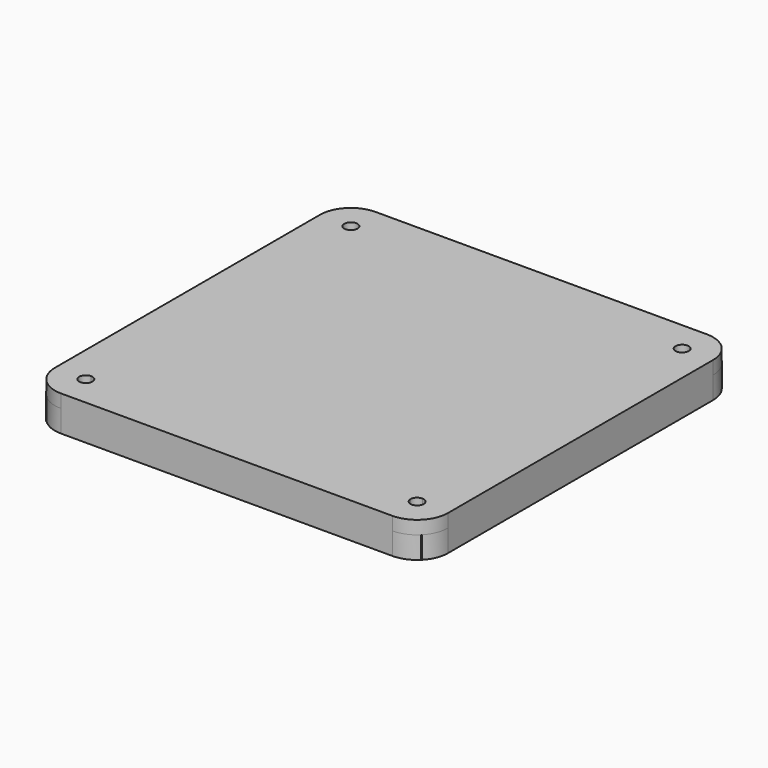
from build123d import *

# Parameters (mm, degrees)
F1_DEPTH = 3
F2_R     = 1.5
F2_W     = 1
F2_H     = 15
F2_W_2   = 9
F2_H_2   = 1
F2_W_3   = 10
F2_H_3   = 10
F2_W_4   = 16
F2_W_5   = 15
F3_DEPTH = 5


with BuildPart() as f1:
    # F0 (on Top) → F1 (new body)
    with BuildSketch(Plane.XY):
        with BuildLine():
            ThreePointArc((-37.5, 44.5), (-32.5502525317, 42.4497474683), (-30.5, 37.5))
            Line((-30.5, 37.5), (30.5, 37.5))
            ThreePointArc((30.5, 37.5), (32.5502525317, 42.4497474683), (37.5, 44.5))
            Line((37.5, 44.5), (-37.5, 44.5))
        make_face()
        with BuildLine():
            Line((30.5, -37.5), (-30.5, -37.5))
            ThreePointArc((-30.5, -37.5), (-32.550252511, -42.4497474476), (-37.4999999416, -44.5))
            Line((-37.4999999416, -44.5), (37.5, -44.5))
            ThreePointArc((37.5, -44.5), (32.5502525317, -42.4497474683), (30.5, -37.5))
        make_face()
        with BuildLine():
            ThreePointArc((44.5, 37.5), (42.4497474683, 32.5502525317), (37.5, 30.5))
            Line((37.5, 30.5), (37.5, -30.5))
            ThreePointArc((37.5, -30.5), (42.4497474683, -32.5502525317), (44.5, -37.5))
            Line((44.5, -37.5), (44.5, 37.5))
        make_face()
        with BuildLine():
            Line((-37.5, -30.5), (-37.5, 30.5))
            ThreePointArc((-37.5, 30.5), (-42.4497474683, 32.5502525317), (-44.5, 37.5))
            Line((-44.5, 37.5), (-44.5, -37.4999999639))
            ThreePointArc((-44.5, -37.4999999639), (-42.4497474555, -32.5502525189), (-37.5, -30.5))
        make_face()
        with BuildLine():
            ThreePointArc((37.5, 44.5), (32.5502525317, 42.4497474683), (30.5, 37.5))
            Line((30.5, 37.5), (36, 37.5))
            ThreePointArc((36, 37.5), (37.5, 39), (39, 37.5))
            ThreePointArc((39, 37.5), (38.5606601718, 36.4393398282), (37.5, 36))
            Line((37.5, 36), (37.5, 30.5))
            ThreePointArc((37.5, 30.5), (42.4497474683, 32.5502525317), (44.5, 37.5))
            ThreePointArc((44.5, 37.5), (42.4497474683, 42.4497474683), (37.5, 44.5))
        make_face()
        with BuildLine():
            Line((-36, 37.5), (-30.5, 37.5))
            ThreePointArc((-30.5, 37.5), (-32.5502525317, 42.4497474683), (-37.5, 44.5))
            ThreePointArc((-37.5, 44.5), (-42.4497474683, 42.4497474683), (-44.5, 37.5))
            ThreePointArc((-44.5, 37.5), (-42.4497474683, 32.5502525317), (-37.5, 30.5))
            Line((-37.5, 30.5), (-37.5, 36))
            ThreePointArc((-37.5, 36), (-38.5606601718, 38.5606601718), (-36, 37.5))
        make_face()
        with BuildLine():
            ThreePointArc((44.5, -37.5), (42.4497474683, -32.5502525317), (37.5, -30.5))
            Line((37.5, -30.5), (37.5, -36))
            ThreePointArc((37.5, -36), (38.5606601718, -36.4393398282), (39, -37.5))
            ThreePointArc((39, -37.5), (37.5, -39), (36, -37.5))
            Line((36, -37.5), (30.5, -37.5))
            ThreePointArc((30.5, -37.5), (32.5502525317, -42.4497474683), (37.5, -44.5))
            ThreePointArc((37.5, -44.5), (42.4497474683, -42.4497474683), (44.5, -37.5))
        make_face()
        with BuildLine():
            Line((-37.5, -36), (-37.5, -30.5))
            ThreePointArc((-37.5, -30.5), (-42.4497474555, -32.5502525189), (-44.5, -37.4999999639))
            ThreePointArc((-44.5, -37.4999999639), (-42.4497474604, -42.4497474762), (-37.4999999416, -44.5))
            ThreePointArc((-37.4999999416, -44.5), (-32.550252511, -42.4497474476), (-30.5, -37.5))
            Line((-30.5, -37.5), (-36, -37.5))
            ThreePointArc((-36, -37.5), (-38.5606601718, -38.5606601718), (-37.5, -36))
        make_face()
        with BuildLine():
            Line((30.5, 37.5), (-30.5, 37.5))
            ThreePointArc((-30.5, 37.5), (-32.5502525317, 32.5502525317), (-37.5, 30.5))
            Line((-37.5, 30.5), (-37.5, -30.5))
            ThreePointArc((-37.5, -30.5), (-32.5502525317, -32.5502525317), (-30.5, -37.5))
            Line((-30.5, -37.5), (30.5, -37.5))
            ThreePointArc((30.5, -37.5), (32.5502525317, -32.5502525317), (37.5, -30.5))
            Line((37.5, -30.5), (37.5, 30.5))
            ThreePointArc((37.5, 30.5), (32.5502525317, 32.5502525317), (30.5, 37.5))
        make_face()
        with BuildLine():
            ThreePointArc((-37.5, 30.5), (-32.5502525317, 32.5502525317), (-30.5, 37.5))
            Line((-30.5, 37.5), (-36, 37.5))
            ThreePointArc((-36, 37.5), (-36.4393398282, 36.4393398282), (-37.5, 36))
            Line((-37.5, 36), (-37.5, 30.5))
        make_face()
        with BuildLine():
            Line((36, 37.5), (30.5, 37.5))
            ThreePointArc((30.5, 37.5), (32.5502525317, 32.5502525317), (37.5, 30.5))
            Line((37.5, 30.5), (37.5, 36))
            ThreePointArc((37.5, 36), (36.4393398282, 36.4393398282), (36, 37.5))
        make_face()
        with BuildLine():
            Line((37.5, -36), (37.5, -30.5))
            ThreePointArc((37.5, -30.5), (32.5502525317, -32.5502525317), (30.5, -37.5))
            Line((30.5, -37.5), (36, -37.5))
            ThreePointArc((36, -37.5), (36.4393398282, -36.4393398282), (37.5, -36))
        make_face()
        with BuildLine():
            ThreePointArc((-30.5, -37.5), (-32.5502525317, -32.5502525317), (-37.5, -30.5))
            Line((-37.5, -30.5), (-37.5, -36))
            ThreePointArc((-37.5, -36), (-36.4393398282, -36.4393398282), (-36, -37.5))
            Line((-36, -37.5), (-30.5, -37.5))
        make_face()
    extrude(amount=F1_DEPTH)

    # F2 (on face) → F3 (join)
    with BuildSketch(Plane(origin=(0, 0, 0), x_dir=(1, 0, 0), z_dir=(0, 0, -1))):
        with BuildLine():
            Line((42.5, 42.3989794856), (42.5, 42.5))
            Line((42.5, 42.5), (42.3989794856, 42.5))
            ThreePointArc((42.3989794856, 42.5), (42.4497474683, 42.4497474683), (42.5, 42.3989794856))
        make_face()
        with BuildLine():
            ThreePointArc((42.5, 42.3989794856), (42.4497474683, 42.4497474683), (42.3989794856, 42.5))
            Line((42.3989794856, 42.5), (37.5, 42.5))
            ThreePointArc((37.5, 42.5), (41.0355339059, 41.0355339059), (42.5, 37.5))
            Line((42.5, 37.5), (42.5, 42.3989794856))
        make_face()
        with BuildLine():
            Line((37.5, 42.5), (42.3989794856, 42.5))
            ThreePointArc((42.3989794856, 42.5), (40.1457513111, 43.9807406984), (37.5, 44.5))
            ThreePointArc((37.5, 44.5), (34.8542486889, 43.9807406984), (32.6010205144, 42.5))
            Line((32.6010205144, 42.5), (37.5, 42.5))
        make_face()
        with BuildLine():
            ThreePointArc((44.5, 37.5), (43.9807406984, 40.1457513111), (42.5, 42.3989794856))
            Line((42.5, 42.3989794856), (42.5, 37.5))
            Line((42.5, 37.5), (42.5, 32.6010205144))
            ThreePointArc((42.5, 32.6010205144), (43.9807406984, 34.8542486889), (44.5, 37.5))
        make_face()
        with BuildLine():
            ThreePointArc((42.5, 37.5), (33.9644660941, 33.9644660941), (37.5, 42.5))
            Line((37.5, 42.5), (32.6010205144, 42.5))
            ThreePointArc((32.6010205144, 42.5), (32.5502525317, 32.5502525317), (42.5, 32.6010205144))
            Line((42.5, 32.6010205144), (42.5, 37.5))
        make_face()
        with BuildLine():
            ThreePointArc((42.5, 37.5), (41.0355339059, 41.0355339059), (37.5, 42.5))
            ThreePointArc((37.5, 42.5), (33.9644660941, 33.9644660941), (42.5, 37.5))
        make_face()
        with Locations((37.5, 37.5)):
            Circle(F2_R, mode=Mode.SUBTRACT)
        with BuildLine():
            ThreePointArc((32.6010205144, 42.5), (34.8542486889, 43.9807406984), (37.5, 44.5))
            Line((37.5, 44.5), (-37.4999999416, 44.5))
            ThreePointArc((-37.4999999416, 44.5), (-34.8542486619, 43.9807406874), (-32.6010205144, 42.5))
            Line((-32.6010205144, 42.5), (32.6010205144, 42.5))
        make_face()
        with BuildLine():
            Line((44.5, -37.5), (44.5, 37.5))
            ThreePointArc((44.5, 37.5), (43.9807406984, 34.8542486889), (42.5, 32.6010205144))
            Line((42.5, 32.6010205144), (42.5, -32.6010205144))
            ThreePointArc((42.5, -32.6010205144), (43.9807406984, -34.8542486889), (44.5, -37.5))
        make_face()
        with BuildLine():
            ThreePointArc((-32.6010205144, 42.5), (-34.8542486619, 43.9807406874), (-37.4999999416, 44.5))
            ThreePointArc((-37.4999999416, 44.5), (-40.145751284, 43.9807407095), (-42.3989794856, 42.5))
            Line((-42.3989794856, 42.5), (-37.5, 42.5))
            Line((-37.5, 42.5), (-32.6010205144, 42.5))
        make_face()
        with BuildLine():
            ThreePointArc((42.5, -42.3989794856), (43.9807406984, -40.1457513111), (44.5, -37.5))
            ThreePointArc((44.5, -37.5), (43.9807406984, -34.8542486889), (42.5, -32.6010205144))
            Line((42.5, -32.6010205144), (42.5, -37.5))
            Line((42.5, -37.5), (42.5, -42.3989794856))
        make_face()
        with BuildLine():
            ThreePointArc((-30.5, 37.5), (-31.0465956117, 40.2117470016), (-32.6010205144, 42.5))
            Line((-32.6010205144, 42.5), (-37.5, 42.5))
            ThreePointArc((-37.5, 42.5), (-33.9644660941, 41.0355339059), (-32.5, 37.5))
            ThreePointArc((-32.5, 37.5), (-37.5, 32.5), (-42.5, 37.5))
            Line((-42.5, 37.5), (-42.5, 32.6010205144))
            ThreePointArc((-42.5, 32.6010205144), (-34.8542486889, 31.0192593016), (-30.5, 37.5))
        make_face()
        with BuildLine():
            ThreePointArc((-42.5, 42.3989794856), (-42.4497474683, 42.4497474683), (-42.3989794856, 42.5))
            Line((-42.3989794856, 42.5), (-42.5, 42.5))
            Line((-42.5, 42.5), (-42.5, 42.3989794856))
        make_face()
        with BuildLine():
            Line((-37.5, 42.5), (-42.3989794856, 42.5))
            ThreePointArc((-42.3989794856, 42.5), (-42.4497474683, 42.4497474683), (-42.5, 42.3989794856))
            Line((-42.5, 42.3989794856), (-42.5, 37.5))
            ThreePointArc((-42.5, 37.5), (-41.0355339059, 41.0355339059), (-37.5, 42.5))
        make_face()
        with BuildLine():
            Line((42.5, -37.5), (42.5, -32.6010205144))
            ThreePointArc((42.5, -32.6010205144), (32.5502525317, -32.5502525317), (32.6010205144, -42.5))
            Line((32.6010205144, -42.5), (37.5, -42.5))
            ThreePointArc((37.5, -42.5), (33.9644660941, -33.9644660941), (42.5, -37.5))
        make_face()
        with BuildLine():
            ThreePointArc((42.3989794856, -42.5), (42.4497474683, -42.4497474683), (42.5, -42.3989794856))
            Line((42.5, -42.3989794856), (42.5, -37.5))
            ThreePointArc((42.5, -37.5), (41.0355339059, -41.0355339059), (37.5, -42.5))
            Line((37.5, -42.5), (42.3989794856, -42.5))
        make_face()
        with BuildLine():
            Line((42.5, -42.5), (42.5, -42.3989794856))
            ThreePointArc((42.5, -42.3989794856), (42.4497474683, -42.4497474683), (42.3989794856, -42.5))
            Line((42.3989794856, -42.5), (42.5, -42.5))
        make_face()
        with BuildLine():
            ThreePointArc((-32.5, 37.5), (-33.9644660941, 41.0355339059), (-37.5, 42.5))
            ThreePointArc((-37.5, 42.5), (-41.0355339059, 41.0355339059), (-42.5, 37.5))
            ThreePointArc((-42.5, 37.5), (-37.5, 32.5), (-32.5, 37.5))
        make_face()
        with Locations((-37.5, 37.5)):
            Circle(F2_R, mode=Mode.SUBTRACT)
        with BuildLine():
            Line((-42.5, 37.5), (-42.5, 42.3989794856))
            ThreePointArc((-42.5, 42.3989794856), (-43.9807407052, 40.1457512943), (-44.5, 37.4999999639))
            ThreePointArc((-44.5, 37.4999999639), (-43.9807406916, 34.8542486722), (-42.5, 32.6010205144))
            Line((-42.5, 32.6010205144), (-42.5, 37.5))
        make_face()
        with BuildLine():
            ThreePointArc((37.5, -42.5), (41.0355339059, -41.0355339059), (42.5, -37.5))
            ThreePointArc((42.5, -37.5), (33.9644660941, -33.9644660941), (37.5, -42.5))
        make_face()
        with Locations((37.5, -37.5)):
            Circle(F2_R, mode=Mode.SUBTRACT)
        with BuildLine():
            ThreePointArc((37.5, -44.5), (34.8542486889, -43.9807406984), (32.6010205144, -42.5))
            Line((32.6010205144, -42.5), (-32.6010205144, -42.5))
            ThreePointArc((-32.6010205144, -42.5), (-34.8542486889, -43.9807406984), (-37.5, -44.5))
            Line((-37.5, -44.5), (37.5, -44.5))
        make_face()
        with BuildLine():
            Line((37.5, -42.5), (32.6010205144, -42.5))
            ThreePointArc((32.6010205144, -42.5), (34.8542486889, -43.9807406984), (37.5, -44.5))
            ThreePointArc((37.5, -44.5), (40.1457513111, -43.9807406984), (42.3989794856, -42.5))
            Line((42.3989794856, -42.5), (37.5, -42.5))
        make_face()
        with BuildLine():
            Line((-42.5, -32.6010205144), (-42.5, 32.6010205144))
            ThreePointArc((-42.5, 32.6010205144), (-43.9807406916, 34.8542486722), (-44.5, 37.4999999639))
            Line((-44.5, 37.4999999639), (-44.5, -37.5))
            ThreePointArc((-44.5, -37.5), (-43.9807406984, -34.8542486889), (-42.5, -32.6010205144))
        make_face()
        with BuildLine():
            ThreePointArc((-37.5, -44.5), (-34.8542486889, -43.9807406984), (-32.6010205144, -42.5))
            Line((-32.6010205144, -42.5), (-37.5, -42.5))
            Line((-37.5, -42.5), (-42.3989794856, -42.5))
            ThreePointArc((-42.3989794856, -42.5), (-40.1457513111, -43.9807406984), (-37.5, -44.5))
        make_face()
        with BuildLine():
            Line((-37.5, -42.5), (-32.6010205144, -42.5))
            ThreePointArc((-32.6010205144, -42.5), (-31.0465956117, -40.2117470016), (-30.5, -37.5))
            ThreePointArc((-30.5, -37.5), (-34.8542486889, -31.0192593016), (-42.5, -32.6010205144))
            Line((-42.5, -32.6010205144), (-42.5, -37.5))
            ThreePointArc((-42.5, -37.5), (-37.5, -32.5), (-32.5, -37.5))
            ThreePointArc((-32.5, -37.5), (-33.9644660941, -41.0355339059), (-37.5, -42.5))
        make_face()
        with BuildLine():
            Line((-42.5, -37.5), (-42.5, -32.6010205144))
            ThreePointArc((-42.5, -32.6010205144), (-43.9807406984, -34.8542486889), (-44.5, -37.5))
            ThreePointArc((-44.5, -37.5), (-43.9807406984, -40.1457513111), (-42.5, -42.3989794856))
            Line((-42.5, -42.3989794856), (-42.5, -37.5))
        make_face()
        with BuildLine():
            Line((-42.3989794856, -42.5), (-37.5, -42.5))
            ThreePointArc((-37.5, -42.5), (-41.0355339059, -41.0355339059), (-42.5, -37.5))
            Line((-42.5, -37.5), (-42.5, -42.3989794856))
            ThreePointArc((-42.5, -42.3989794856), (-42.4497474683, -42.4497474683), (-42.3989794856, -42.5))
        make_face()
        with BuildLine():
            ThreePointArc((-42.5, -37.5), (-41.0355339059, -41.0355339059), (-37.5, -42.5))
            ThreePointArc((-37.5, -42.5), (-33.9644660941, -41.0355339059), (-32.5, -37.5))
            ThreePointArc((-32.5, -37.5), (-37.5, -32.5), (-42.5, -37.5))
        make_face()
        with Locations((-37.5, -37.5)):
            Circle(F2_R, mode=Mode.SUBTRACT)
        with BuildLine():
            ThreePointArc((-42.3989794856, -42.5), (-42.4497474683, -42.4497474683), (-42.5, -42.3989794856))
            Line((-42.5, -42.3989794856), (-42.5, -42.5))
            Line((-42.5, -42.5), (-42.3989794856, -42.5))
        make_face()
        with Locations((0, 30)):
            Rectangle(F2_W, F2_H)
        with Locations((5, 22)):
            Rectangle(F2_W_2, F2_H_2)
        with Locations((0, 22)):
            Rectangle(F2_W, F2_H_2)
        with Locations((-5.5, 22)):
            Rectangle(F2_W_3, F2_H_2)
        with Locations((0, 16.5)):
            Rectangle(F2_W, F2_H_3)
        with Locations((10, 30)):
            Rectangle(F2_W, F2_H)
        with Locations((10, 22)):
            Rectangle(F2_W, F2_H_2)
        with Locations((-11, 22)):
            Rectangle(F2_W, F2_H_2)
        with Locations((-11, 30)):
            Rectangle(F2_W, F2_H)
        with Locations((5, 11)):
            Rectangle(F2_W_2, F2_H_2)
        with Locations((0, 11)):
            Rectangle(F2_W, F2_H_2)
        with Locations((10, 16.5)):
            Rectangle(F2_W, F2_H_3)
        with Locations((15.5, 22)):
            Rectangle(F2_W_3, F2_H_2)
        with Locations((-5.5, 11)):
            Rectangle(F2_W_3, F2_H_2)
        with Locations((-11, 16.5)):
            Rectangle(F2_W, F2_H_3)
        with Locations((-16.5, 22)):
            Rectangle(F2_W_3, F2_H_2)
        with Locations((0, 5.5)):
            Rectangle(F2_W, F2_H_3)
        with Locations((10, 11)):
            Rectangle(F2_W, F2_H_2)
        with Locations((21, 22)):
            Rectangle(F2_W, F2_H_2)
        with Locations((21, 30)):
            Rectangle(F2_W, F2_H)
        with Locations((-11, 11)):
            Rectangle(F2_W, F2_H_2)
        with Locations((-22, 30)):
            Rectangle(F2_W, F2_H)
        with Locations((-22, 22)):
            Rectangle(F2_W, F2_H_2)
        with Locations((5, 0)):
            Rectangle(F2_W_2, F2_H_2)
        Rectangle(F2_W, F2_H_2)
        with Locations((10, 5.5)):
            Rectangle(F2_W, F2_H_3)
        with Locations((15.5, 11)):
            Rectangle(F2_W_3, F2_H_2)
        with Locations((21, 16.5)):
            Rectangle(F2_W, F2_H_3)
        with Locations((29.5, 22)):
            Rectangle(F2_W_4, F2_H_2)
        with Locations((-5.5, 0)):
            Rectangle(F2_W_3, F2_H_2)
        with Locations((-11, 5.5)):
            Rectangle(F2_W, F2_H_3)
        with Locations((-16.5, 11)):
            Rectangle(F2_W_3, F2_H_2)
        with Locations((-22, 16.5)):
            Rectangle(F2_W, F2_H_3)
        with Locations((-30, 22)):
            Rectangle(F2_W_5, F2_H_2)
        with Locations((0, -5.5)):
            Rectangle(F2_W, F2_H_3)
        with Locations((10, 0)):
            Rectangle(F2_W, F2_H_2)
        with Locations((21, 11)):
            Rectangle(F2_W, F2_H_2)
        with Locations((-11, 0)):
            Rectangle(F2_W, F2_H_2)
        with Locations((-22, 11)):
            Rectangle(F2_W, F2_H_2)
        with Locations((5, -11)):
            Rectangle(F2_W_2, F2_H_2)
        with Locations((0, -11)):
            Rectangle(F2_W, F2_H_2)
        with Locations((10, -5.5)):
            Rectangle(F2_W, F2_H_3)
        with Locations((15.5, 0)):
            Rectangle(F2_W_3, F2_H_2)
        with Locations((21, 5.5)):
            Rectangle(F2_W, F2_H_3)
        with Locations((29.5, 11)):
            Rectangle(F2_W_4, F2_H_2)
        with Locations((-5.5, -11)):
            Rectangle(F2_W_3, F2_H_2)
        with Locations((-11, -5.5)):
            Rectangle(F2_W, F2_H_3)
        with Locations((-16.5, 0)):
            Rectangle(F2_W_3, F2_H_2)
        with Locations((-22, 5.5)):
            Rectangle(F2_W, F2_H_3)
        with Locations((-30, 11)):
            Rectangle(F2_W_5, F2_H_2)
        with Locations((0, -16.5)):
            Rectangle(F2_W, F2_H_3)
        with Locations((10, -11)):
            Rectangle(F2_W, F2_H_2)
        with Locations((21, 0)):
            Rectangle(F2_W, F2_H_2)
        with Locations((-11, -11)):
            Rectangle(F2_W, F2_H_2)
        with Locations((-22, 0)):
            Rectangle(F2_W, F2_H_2)
        with Locations((5, -22)):
            Rectangle(F2_W_2, F2_H_2)
        with Locations((0, -22)):
            Rectangle(F2_W, F2_H_2)
        with Locations((10, -16.5)):
            Rectangle(F2_W, F2_H_3)
        with Locations((15.5, -11)):
            Rectangle(F2_W_3, F2_H_2)
        with Locations((21, -5.5)):
            Rectangle(F2_W, F2_H_3)
        with Locations((29.5, 0)):
            Rectangle(F2_W_4, F2_H_2)
        with Locations((-5.5, -22)):
            Rectangle(F2_W_3, F2_H_2)
        with Locations((-11, -16.5)):
            Rectangle(F2_W, F2_H_3)
        with Locations((-16.5, -11)):
            Rectangle(F2_W_3, F2_H_2)
        with Locations((-22, -5.5)):
            Rectangle(F2_W, F2_H_3)
        with Locations((-30, 0)):
            Rectangle(F2_W_5, F2_H_2)
        with Locations((0, -30)):
            Rectangle(F2_W, F2_H)
        with Locations((10, -22)):
            Rectangle(F2_W, F2_H_2)
        with Locations((21, -11)):
            Rectangle(F2_W, F2_H_2)
        with Locations((-11, -22)):
            Rectangle(F2_W, F2_H_2)
        with Locations((-22, -11)):
            Rectangle(F2_W, F2_H_2)
        with Locations((10, -30)):
            Rectangle(F2_W, F2_H)
        with Locations((15.5, -22)):
            Rectangle(F2_W_3, F2_H_2)
        with Locations((21, -16.5)):
            Rectangle(F2_W, F2_H_3)
        with Locations((29.5, -11)):
            Rectangle(F2_W_4, F2_H_2)
        with Locations((-11, -30)):
            Rectangle(F2_W, F2_H)
        with Locations((-16.5, -22)):
            Rectangle(F2_W_3, F2_H_2)
        with Locations((-22, -16.5)):
            Rectangle(F2_W, F2_H_3)
        with Locations((-30, -11)):
            Rectangle(F2_W_5, F2_H_2)
        with Locations((21, -22)):
            Rectangle(F2_W, F2_H_2)
        with Locations((-22, -22)):
            Rectangle(F2_W, F2_H_2)
        with Locations((21, -30)):
            Rectangle(F2_W, F2_H)
        with Locations((29.5, -22)):
            Rectangle(F2_W_4, F2_H_2)
        with Locations((-22, -30)):
            Rectangle(F2_W, F2_H)
        with Locations((-30, -22)):
            Rectangle(F2_W_5, F2_H_2)
    extrude(amount=F3_DEPTH)


solid = f1.part
